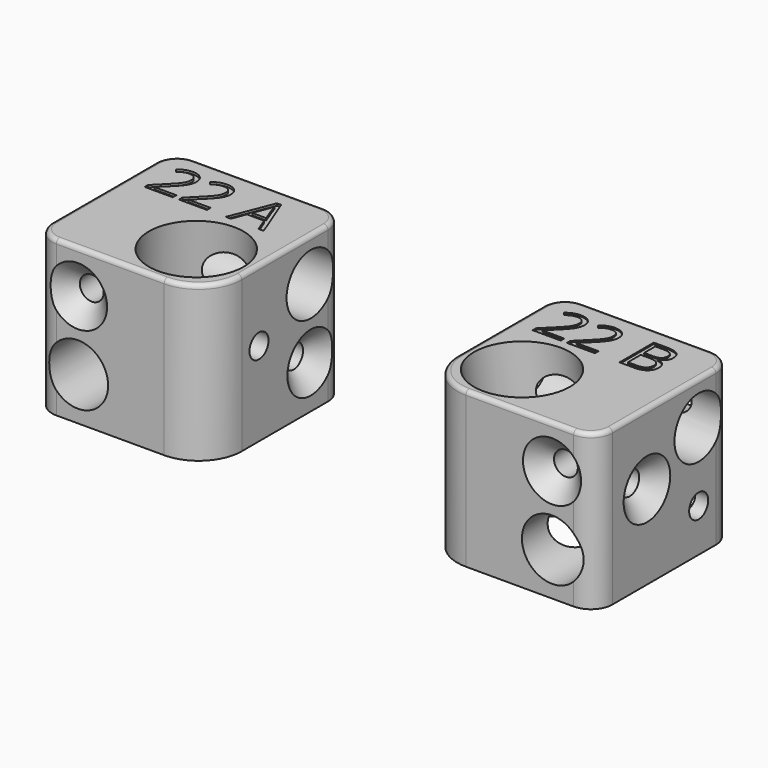
from build123d import *

# Parameters (mm, degrees)
F4_W          = 40
F4_H          = 40
F5_DEPTH      = 36
F6_R          = 11
F7_DEPTH      = 75
F8_R          = 7
F8_R_2        = 2.7625
F9_DEPTH      = 40.001
F10_R         = 7
F10_R_2       = 2.7625
F11_DEPTH     = 40.001
F12_R         = 10
F13_T1_DEPTH  = 61
F14_R         = 1
F19_TEXT_SIZE = 13.8888888889
F20_DEPTH     = 0.5
F21_TEXT_SIZE = 13.8888888889
F22_DEPTH     = 0.3


# Not quite as in the source:
# - a fillet or chamfer that OpenCascade refuses, or shapes differently, is made with other operations: its cross-section is extruded or revolved along the edge and cut away or added
# - Text() gives the source's letters only with a copy of the font that has no kerning and outlines rounded to 1/6400 em; it was checked with that copy


with BuildPart() as f5:
    # F4 (on Top) → F5 (new body)
    with BuildSketch(Plane.XY):
        Rectangle(F4_W, F4_H)
    extrude(amount=F5_DEPTH)

    # F6 (on line) → F7 (cut, symmetric)
    with BuildSketch(Plane(origin=(0, 0, 0), x_dir=(0.9962800468, 0.0074537962, -0.0858516706), z_dir=(-0.0861746391, 0.0861746391, -0.9925461516))):
        with Locations((4.0445826283, 4.0749567379)):
            Circle(F6_R)
    extrude(amount=F7_DEPTH, both=True, mode=Mode.SUBTRACT)

    # F8 (on face) → F9 (cut, through all)
    with BuildSketch(Plane.YZ.offset(20)):
        with Locations((10, 26)):
            Circle(F8_R)
        with Locations((10, 10)):
            Circle(F8_R_2)
        with Locations((-5, 19.5)):
            Circle(F8_R_2)
    extrude(amount=-F9_DEPTH, mode=Mode.SUBTRACT)

    # F10 (on face) → F11 (cut, through all)
    with BuildSketch(Plane(origin=(0, 20, 0), x_dir=(-1, 0, 0), z_dir=(0, 1, 0))):
        with Locations((10, 10)):
            Circle(F10_R)
        with Locations((10, 26)):
            Circle(F10_R_2)
    extrude(amount=-F11_DEPTH, mode=Mode.SUBTRACT)

    # F12
    f12_edges = [f5.edges().sort_by_distance(p)[0] for p in [
        (20, -20, 18),
    ]]
    fillet(f12_edges, radius=F12_R)

    # F13: fillet of radius 5 on 3 edges, made by hand

    # F13_s2 → F13_t1 (cut)
    with BuildSketch(Plane.XY.offset(-12.5)):
        with BuildLine():
            ThreePointArc((-15, -20), (-18.5355339059, -18.5355339059), (-20, -15))
            Line((-20, -15), (-20, -20))
            Line((-20, -20), (-15, -20))
        make_face()
        with BuildLine():
            ThreePointArc((-20, 15), (-18.5355339059, 18.5355339059), (-15, 20))
            Line((-15, 20), (-20, 20))
            Line((-20, 20), (-20, 15))
        make_face()
        with BuildLine():
            ThreePointArc((20, 15), (18.5355339059, 18.5355339059), (15, 20))
            Line((15, 20), (20, 20))
            Line((20, 20), (20, 15))
        make_face()
    extrude(amount=F13_T1_DEPTH, mode=Mode.SUBTRACT)

    # F14
    f14_edges = [f5.edges().sort_by_distance(p)[0] for p in [
        (20, 2.5, 36),
        (-2.5, -20, 36),
        (17.071068, -17.071068, 36),
        (-18.535534, -18.535534, 36),
        (-20, 0, 36),
        (-18.535534, 18.535534, 36),
        (0, 20, 36),
        (18.535534, 18.535534, 36),
    ]]
    fillet(f14_edges, radius=F14_R)

    # F15: chamfer of 4 on 3 edges, made by hand

    # F15_s1 → F15_t2 (revolve, cut)
    with BuildSketch(Plane.XY.offset(26)):
        Polygon((-16.7625, -20), (-12.7625, -16), (-12.7625, -20), align=None)
    revolve(axis=Axis((-10, -20, 26), (0, 1, 0)), mode=Mode.SUBTRACT)

    # F15_s3 → F15_t4 (revolve, cut)
    with BuildSketch(Plane.XY.offset(19.5)):
        Polygon((-20, 1.7625), (-16, -2.2375), (-20, -2.2375), align=None)
    revolve(axis=Axis((-20, -5, 19.5), (1, 0, 0)), mode=Mode.SUBTRACT)

    # F15_s5 → F15_t6 (revolve, cut)
    with BuildSketch(Plane.XY.offset(10)):
        Polygon((20, 16.7625), (16, 12.7625), (20, 12.7625), align=None)
    revolve(axis=Axis((20, 10, 10), (1, 0, 0)), mode=Mode.SUBTRACT)


with BuildPart() as f17_1:
    # F17: instance of F5
    add(f5.part.mirror(Plane(origin=(45, -0.4885641497, 17.0728724101), x_dir=(0, 1, 0), z_dir=(1, 0, 0))))

    # F21 (on face) → F22 (cut)
    with BuildSketch(Plane.XY.offset(36)):
        with Locations((74, 6)):
            Text('22 B', F21_TEXT_SIZE, font='Open Sans', text_align=(TextAlign.LEFT, TextAlign.BOTTOM))
    extrude(amount=-F22_DEPTH, mode=Mode.SUBTRACT)


with BuildPart() as f5_1:
    add(f5.part)

    # F19 (on face) → F20 (cut)
    with BuildSketch(Plane.XY.offset(36)):
        with Locations((-16, 6)):
            Text('22 A', F19_TEXT_SIZE, font='Open Sans', text_align=(TextAlign.LEFT, TextAlign.BOTTOM))
    extrude(amount=-F20_DEPTH, mode=Mode.SUBTRACT)


solid = Compound([f17_1.part, f5_1.part])
